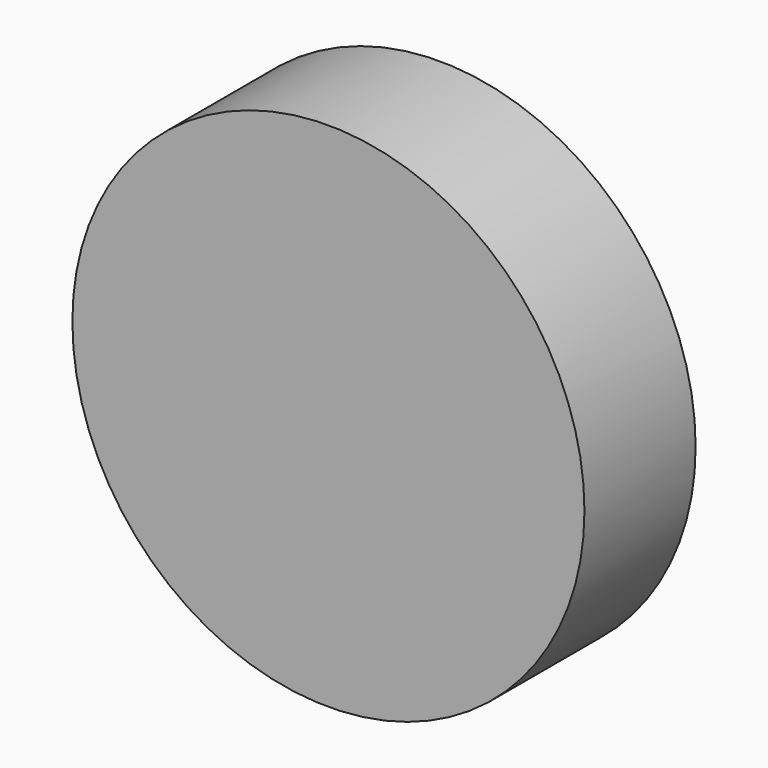
from build123d import *

# Parameters (mm, degrees)
F0_R     = 46.8022742285
F1_DEPTH = 25.4


# Not quite as in the source:
# - the program builds the solid bodies; features that only make, move or delete a surface that nothing else refers to are left out


with BuildPart() as f1:
    # F0 (on Front) → F1 (new body)
    with BuildSketch(Plane.XZ):
        Circle(F0_R)
    extrude(amount=F1_DEPTH)


solid = f1.part
